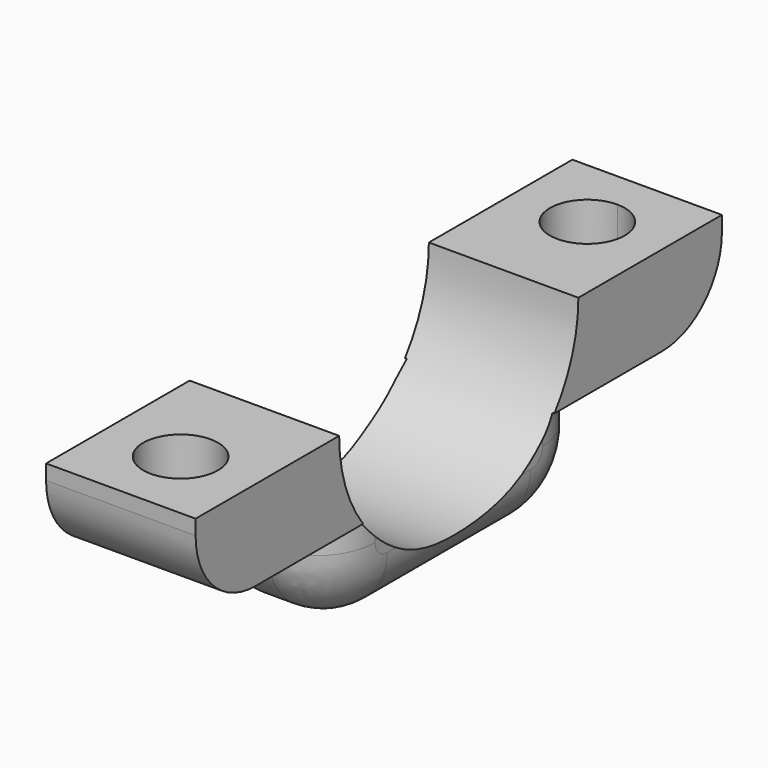
from build123d import *

# Parameters (mm, degrees)
F0_W          = 12.7
F0_H          = 3.175
F0_H_2        = 12.7
F1_DEPTH      = 27.94
F2_W          = 12.7
F2_H          = 10.9347
F2_H_2        = 3.0353
F3_DEPTH      = 7.62
F4_W          = 12.7
F4_H          = 13.97
F5_DEPTH      = 7.62
F7_DEPTH      = 25.4
F10_DEPTH     = 25.4
F11_T1_DEPTH  = 44.45
F12_R         = 6.35
F13_R         = 6.35
F14_T1_DEPTH  = 15.24
F14_T3_DEPTH  = 1.905
F14_T6_ANGLE  = 90
F14_T8_ANGLE  = 90
F14_T10_ANGLE = 90
F14_T12_ANGLE = 90


# Not quite as in the source:
# - a fillet or chamfer that OpenCascade refuses, or shapes differently, is made with other operations: its cross-section is extruded or revolved along the edge and cut away or added


with BuildPart() as f1:
    # F0 (on Front) → F1 (new body)
    with BuildSketch(Plane.XZ):
        with Locations((-19.05, 11.1125)):
            Rectangle(F0_W, F0_H)
        with Locations((-19.05, 19.05)):
            Rectangle(F0_W, F0_H_2)
    extrude(amount=F1_DEPTH)

    # F2 (on face) → F3 (join)
    with BuildSketch(Plane.XY.offset(25.4)):
        with Locations((-19.05, -33.40735)):
            Rectangle(F2_W, F2_H)
        with Locations((-19.05, -40.39235)):
            Rectangle(F2_W, F2_H_2)
    extrude(amount=-F3_DEPTH)

    # F4 (on face) → F5 (join)
    with BuildSketch(Plane.XY.offset(25.4)):
        with Locations((-19.05, 6.985)):
            Rectangle(F4_W, F4_H)
    extrude(amount=-F5_DEPTH)

    # F6 (on face) → F7 (cut)
    with BuildSketch(Plane(origin=(-25.4, 0, 0), x_dir=(0, -1, 0), z_dir=(-1, 0, 0))):
        with BuildLine():
            ThreePointArc((1.27, 25.4), (13.97, 12.7), (26.67, 25.4))
            Line((26.67, 25.4), (1.27, 25.4))
        make_face()
    extrude(amount=-F7_DEPTH, mode=Mode.SUBTRACT)

    # F8 (on face) + F9 (on face) → F10 (cut)
    with BuildSketch(Plane(origin=(0, 0, 17.78), x_dir=(1, 0, 0), z_dir=(0, 0, -1))):
        with BuildLine():
            ThreePointArc((-19.05, 38.735), (-21.2950640303, 33.3149359697), (-15.875, 35.56))
            ThreePointArc((-15.875, 35.56), (-16.8049359697, 37.8050640303), (-19.05, 38.735))
        make_face()
    with BuildSketch(Plane(origin=(0, 0, 17.78), x_dir=(1, 0, 0), z_dir=(0, 0, -1))):
        with BuildLine():
            ThreePointArc((-19.05, -10.795), (-16.8049359697, -9.8650640303), (-15.875, -7.62))
            ThreePointArc((-15.875, -7.62), (-21.2950640303, -5.3749359697), (-19.05, -10.795))
        make_face()
    extrude(amount=-F10_DEPTH, mode=Mode.SUBTRACT)

    # F11: fillet of radius 6.35 on 2 edges, made by hand

    # F11_s2 → F11_t1 (cut)
    with BuildSketch(Plane.YZ.offset(-41.275)):
        with BuildLine():
            ThreePointArc((-35.56, 17.78), (-40.0501280605, 19.6398719395), (-41.91, 24.13))
            Line((-41.91, 24.13), (-41.91, 17.78))
            Line((-41.91, 17.78), (-35.56, 17.78))
        make_face()
        with BuildLine():
            ThreePointArc((13.97, 24.13), (12.1101280605, 19.6398719395), (7.62, 17.78))
            Line((7.62, 17.78), (13.97, 17.78))
            Line((13.97, 17.78), (13.97, 24.13))
        make_face()
    extrude(amount=F11_T1_DEPTH, mode=Mode.SUBTRACT)

    # F12
    f12_edges = [f1.edges().sort_by_distance(p)[0] for p in [
        (-19.05, 0, 9.525),
    ]]
    fillet(f12_edges, radius=F12_R)

    # F13
    f13_edges = [f1.edges().sort_by_distance(p)[0] for p in [
        (-19.05, -27.94, 9.525),
    ]]
    fillet(f13_edges, radius=F13_R)

    # F14: fillet of radius 5.08 on 2 edges, made by hand

    # F14_s2 → F14_t1 (cut)
    with BuildSketch(Plane.XZ.offset(6.35)):
        with BuildLine():
            ThreePointArc((-17.78, 9.525), (-14.1878975516, 11.0128975516), (-12.7, 14.605))
            Line((-12.7, 14.605), (-12.7, 9.525))
            Line((-12.7, 9.525), (-17.78, 9.525))
        make_face()
        with BuildLine():
            ThreePointArc((-20.32, 9.525), (-23.9121024484, 11.0128975516), (-25.4, 14.605))
            Line((-25.4, 14.605), (-25.4, 9.525))
            Line((-25.4, 9.525), (-20.32, 9.525))
        make_face()
    extrude(amount=F14_T1_DEPTH, mode=Mode.SUBTRACT)

    # F14_s4 → F14_t3 (cut)
    with BuildSketch(Plane.XY.offset(15.875)):
        with BuildLine():
            ThreePointArc((-25.4, -22.86), (-23.9121024484, -26.4521024484), (-20.32, -27.94))
            Line((-20.32, -27.94), (-25.4, -27.94))
            Line((-25.4, -27.94), (-25.4, -22.86))
        make_face()
        with BuildLine():
            ThreePointArc((-25.4, -5.08), (-23.9121024484, -1.4878975516), (-20.32, 0))
            Line((-20.32, 0), (-25.4, 0))
            Line((-25.4, 0), (-25.4, -5.08))
        make_face()
        with BuildLine():
            ThreePointArc((-12.7, -22.86), (-14.1878975516, -26.4521024484), (-17.78, -27.94))
            Line((-17.78, -27.94), (-12.7, -27.94))
            Line((-12.7, -27.94), (-12.7, -22.86))
        make_face()
        with BuildLine():
            ThreePointArc((-12.7, -5.08), (-14.1878975516, -1.4878975516), (-17.78, 0))
            Line((-17.78, 0), (-12.7, 0))
            Line((-12.7, 0), (-12.7, -5.08))
        make_face()
    extrude(amount=F14_T3_DEPTH, mode=Mode.SUBTRACT)

    # F14_s5 → F14_t6 (revolve, cut)
    with BuildSketch(Plane.XZ.offset(6.35)):
        with BuildLine():
            ThreePointArc((-25.4, 14.605), (-23.9121024484, 11.0128975516), (-20.32, 9.525))
            Line((-20.32, 9.525), (-25.4, 9.525))
            Line((-25.4, 9.525), (-25.4, 14.605))
        make_face()
    revolve(axis=Axis((-25.4, -6.35, 15.875), (1, 0, 0)), revolution_arc=F14_T6_ANGLE, mode=Mode.SUBTRACT)

    # F14_s7 → F14_t8 (revolve, cut)
    with BuildSketch(Plane.XZ.offset(21.59)):
        with BuildLine():
            ThreePointArc((-25.4, 14.605), (-23.9121024484, 11.0128975516), (-20.32, 9.525))
            Line((-20.32, 9.525), (-25.4, 9.525))
            Line((-25.4, 9.525), (-25.4, 14.605))
        make_face()
    revolve(axis=Axis((-25.4, -21.59, 15.875), (-1, 0, 0)), revolution_arc=F14_T8_ANGLE, mode=Mode.SUBTRACT)

    # F14_s9 → F14_t10 (revolve, cut)
    with BuildSketch(Plane.XZ.offset(6.35)):
        with BuildLine():
            ThreePointArc((-17.78, 9.525), (-14.1878975516, 11.0128975516), (-12.7, 14.605))
            Line((-12.7, 14.605), (-12.7, 9.525))
            Line((-12.7, 9.525), (-17.78, 9.525))
        make_face()
    revolve(axis=Axis((-12.7, -6.35, 15.875), (1, 0, 0)), revolution_arc=F14_T10_ANGLE, mode=Mode.SUBTRACT)

    # F14_s11 → F14_t12 (revolve, cut)
    with BuildSketch(Plane.XZ.offset(21.59)):
        with BuildLine():
            ThreePointArc((-17.78, 9.525), (-14.1878975516, 11.0128975516), (-12.7, 14.605))
            Line((-12.7, 14.605), (-12.7, 9.525))
            Line((-12.7, 9.525), (-17.78, 9.525))
        make_face()
    revolve(axis=Axis((-12.7, -21.59, 15.875), (-1, 0, 0)), revolution_arc=F14_T12_ANGLE, mode=Mode.SUBTRACT)


solid = f1.part
